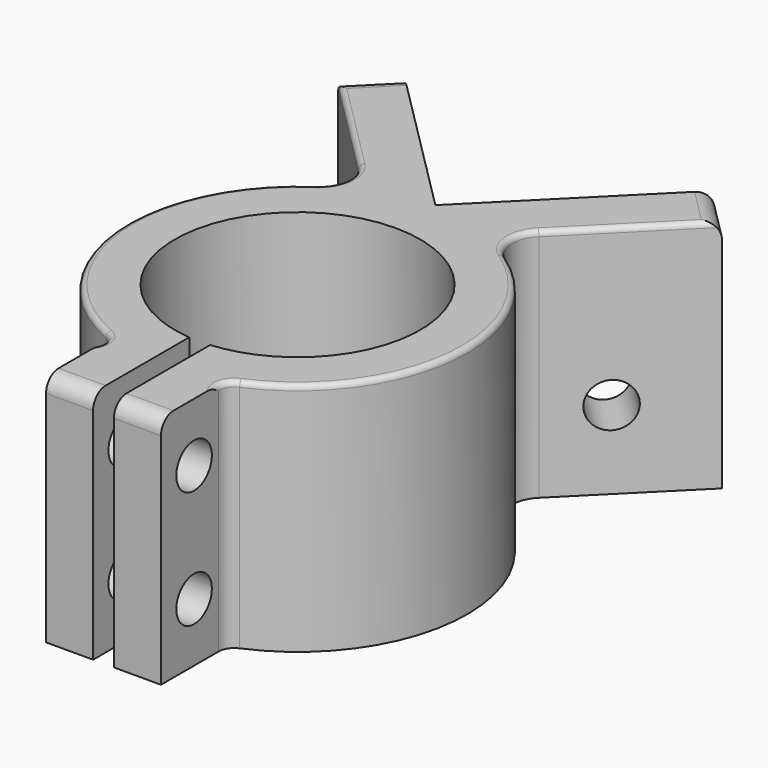
from build123d import *

# Parameters (mm, degrees)
F1_DEPTH      = 45
F2_R          = 4.25
F3_DEPTH      = 10
F4_R          = 4.25
F5_DEPTH      = 10
F6_R          = 4.25
F7_DEPTH      = 22
F9_DEPTH      = 3
F10_R         = 6
F11_T1_DEPTH  = 45
F11_T6_DEPTH  = 50.1024684741
F11_T11_DEPTH = 50.1024684741
F11_T17_DEPTH = 55.2049369483
F11_T23_DEPTH = 50.1024684741
F11_T25_DEPTH = 24
F11_T27_DEPTH = 24
F11_T29_DEPTH = 25
F11_T31_DEPTH = 25
F12_T3_ANGLE  = 122.7559288298
F12_T6_ANGLE  = 114.5305881861
F12_T9_ANGLE  = 100.9823800972
F12_T12_DEPTH = 27.0396198775
F12_T15_DEPTH = 27.0396198775
F12_T18_ANGLE = 100.9823800972
F12_T21_ANGLE = 114.5305881861
F12_T24_ANGLE = 122.7559288298


# Not quite as in the source:
# - a fillet or chamfer that OpenCascade refuses, or shapes differently, is made with other operations: its cross-section is extruded or revolved along the edge and cut away or added


with BuildPart() as f1:
    # F0 (on Top) → F1 (new body)
    with BuildSketch(Plane.XY):
        with BuildLine():
            Line((29.6984848098, 29.6984848098), (0, 0))
            Line((0, 0), (-29.6984848098, 29.6984848098))
            Line((-29.6984848098, 29.6984848098), (-36.7695526217, 22.627416998))
            Line((-36.7695526217, 22.627416998), (-11.5286496808, -2.613485943))
            ThreePointArc((-11.5286496808, -2.613485943), (-32.4987783251, -33.2817931394), (-11, -63.5818573667))
            ThreePointArc((-11, -63.5818573667), (-8.6210949019, -64.3357100238), (-6.1913611889, -64.9048122801))
            Line((-6.1913611889, -64.9048122801), (-9, -54.7082933461))
            ThreePointArc((-9, -54.7082933461), (0, -9.5), (9, -54.7082933461))
            Line((9, -54.7082933461), (6.1913611889, -64.9048122801))
            ThreePointArc((6.1913611889, -64.9048122801), (8.6210949019, -64.3357100238), (11, -63.5818573667))
            ThreePointArc((11, -63.5818573667), (32.4987783251, -33.2817931394), (11.5286496808, -2.613485943))
            Line((11.5286496808, -2.613485943), (36.7695526217, 22.627416998))
            Line((36.7695526217, 22.627416998), (29.6984848098, 29.6984848098))
        make_face()
        with BuildLine():
            ThreePointArc((-6.1913611889, -64.9048122801), (-8.6210949019, -64.3357100238), (-11, -63.5818573667))
            Line((-11, -63.5818573667), (-11, -79.4384031666))
            Line((-11, -79.4384031666), (-2, -79.4384031666))
            Line((-2, -79.4384031666), (-2, -67.4147389479))
            Line((-2, -67.4147389479), (-5.5, -67.4147389479))
            Line((-5.5, -67.4147389479), (-6.1913611889, -64.9048122801))
        make_face()
        with BuildLine():
            Line((11, -79.4384031666), (11, -63.5818573667))
            ThreePointArc((11, -63.5818573667), (8.6210949019, -64.3357100238), (6.1913611889, -64.9048122801))
            Line((6.1913611889, -64.9048122801), (5.5, -67.4147389479))
            Line((5.5, -67.4147389479), (2, -67.4147389479))
            Line((2, -67.4147389479), (2, -79.4384031666))
            Line((2, -79.4384031666), (11, -79.4384031666))
        make_face()
        with BuildLine():
            Line((-9, -54.7082933461), (-6.1913611889, -64.9048122801))
            ThreePointArc((-6.1913611889, -64.9048122801), (-4.1043610148, -65.2397925034), (-2, -65.4384031666))
            Line((-2, -65.4384031666), (-2, -56.4147389479))
            ThreePointArc((-2, -56.4147389479), (-5.565787379, -55.8313821494), (-9, -54.7082933461))
        make_face()
        with BuildLine():
            ThreePointArc((2, -65.4384031666), (4.1043610148, -65.2397925034), (6.1913611889, -64.9048122801))
            Line((6.1913611889, -64.9048122801), (9, -54.7082933461))
            ThreePointArc((9, -54.7082933461), (5.565787379, -55.8313821494), (2, -56.4147389479))
            Line((2, -56.4147389479), (2, -65.4384031666))
        make_face()
        with BuildLine():
            ThreePointArc((-2, -65.4384031666), (-4.1043610148, -65.2397925034), (-6.1913611889, -64.9048122801))
            Line((-6.1913611889, -64.9048122801), (-5.5, -67.4147389479))
            Line((-5.5, -67.4147389479), (-2, -67.4147389479))
            Line((-2, -67.4147389479), (-2, -65.4384031666))
        make_face()
        with BuildLine():
            Line((5.5, -67.4147389479), (6.1913611889, -64.9048122801))
            ThreePointArc((6.1913611889, -64.9048122801), (4.1043610148, -65.2397925034), (2, -65.4384031666))
            Line((2, -65.4384031666), (2, -67.4147389479))
            Line((2, -67.4147389479), (5.5, -67.4147389479))
        make_face()
    extrude(amount=F1_DEPTH)

    # F2 (on face) → F3 (cut, through all)
    with BuildSketch(Plane(origin=(0, 0, 0), x_dir=(-0.7071067812, -0.7071067812, 0), z_dir=(-0.7071067812, 0.7071067812, 0))):
        with Locations((-25.4, 15)):
            Circle(F2_R)
    extrude(amount=-F3_DEPTH, mode=Mode.SUBTRACT)

    # F4 (on face) → F5 (cut, through all)
    with BuildSketch(Plane(origin=(0, 0, 0), x_dir=(-0.7071067812, 0.7071067812, 0), z_dir=(0.7071067812, 0.7071067812, 0))):
        with Locations((25.4, 15)):
            Circle(F4_R)
    extrude(amount=-F5_DEPTH, mode=Mode.SUBTRACT)

    # F6 (on face) → F7 (cut, through all)
    with BuildSketch(Plane.YZ.offset(11)):
        with Locations((-71.5101302667, 33.75)):
            Circle(F6_R)
        with Locations((-71.5101302667, 11.25)):
            Circle(F6_R)
    extrude(amount=-F7_DEPTH, mode=Mode.SUBTRACT)

    # F8 (on face) → F9 (cut)
    with BuildSketch(Plane(origin=(-11, 0, 0), x_dir=(0, -1, 0), z_dir=(-1, 0, 0))):
        Polygon((78.4351302667, 37.7481506141), (71.5101302667, 41.7463012283), (64.5851302667, 37.7481506141), (64.5851302667, 29.7518493859), (71.5101302667, 25.7536987717), (78.4351302667, 29.7518493859), align=None)
        Polygon((71.5101302667, 19.2463012283), (64.5851302667, 15.2481506141), (64.5851302667, 7.2518493859), (71.5101302667, 3.2536987717), (78.4351302667, 7.2518493859), (78.4351302667, 15.2481506141), align=None)
    extrude(amount=-F9_DEPTH, mode=Mode.SUBTRACT)

    # F10
    f10_edges = [f1.edges().sort_by_distance(p)[0] for p in [
        (-11.52865, -2.613486, 22.5),
        (11.52865, -2.613486, 22.5),
    ]]
    fillet(f10_edges, radius=F10_R)

    # F11: fillet of radius 3 on 6 edges, made by hand

    # F11_s2 → F11_t1 (join)
    with BuildSketch(Plane.XY):
        with BuildLine():
            ThreePointArc((12.8169014085, -62.8659846361), (11.4950752731, -63.9719807061), (11, -65.6228447564))
            Line((11, -65.6228447564), (11, -63.5818573667))
            ThreePointArc((11, -63.5818573667), (11.9138287975, -63.2375707256), (12.8169014085, -62.8659846361))
        make_face()
    extrude(amount=F11_T1_DEPTH)


with BuildPart() as f11_tool4:
    # F11_s5 → F11_t6 (new body)
    with BuildSketch(Plane.XY):
        with BuildLine():
            ThreePointArc((-11, -65.6228447564), (-11.4950752731, -63.9719807061), (-12.8169014085, -62.8659846361))
            ThreePointArc((-12.8169014085, -62.8659846361), (-11.9138287975, -63.2375707256), (-11, -63.5818573667))
            Line((-11, -63.5818573667), (-11, -65.6228447564))
        make_face()
    extrude(amount=F11_T6_DEPTH)

    split(bisect_by=Plane(origin=(0, -19.286425463, 33.4050687982), x_dir=(1, 0, 0), z_dir=(0, 0.5, -0.8660254038)), keep=Keep.TOP)


with BuildPart() as f1_1:
    add(f1.part)

    # F11_t3: union F11_tool4
    add(f11_tool4.part)


with BuildPart() as f11_tool9:
    # F11_s10 → F11_t11 (new body)
    with BuildSketch(Plane.XY.offset(-5.1024684741)):
        with BuildLine():
            ThreePointArc((-11, -65.6228447564), (-11.4950752731, -63.9719807061), (-12.8169014085, -62.8659846361))
            ThreePointArc((-12.8169014085, -62.8659846361), (-11.9138287975, -63.2375707256), (-11, -63.5818573667))
            Line((-11, -63.5818573667), (-11, -65.6228447564))
        make_face()
    extrude(amount=F11_T11_DEPTH)

    split(bisect_by=Plane.XZ.offset(64.5851302667), keep=Keep.BOTTOM)

    split(bisect_by=Plane(origin=(0, -19.286425463, 33.4050687982), x_dir=(1, 0, 0), z_dir=(0, -0.5, 0.8660254038)), keep=Keep.TOP)


with BuildPart() as f1_2:
    add(f1_1.part)

    # F11_t8: union F11_tool9
    add(f11_tool9.part)


with BuildPart() as f11_tool15:
    # F11_s16 → F11_t17 (new body)
    with BuildSketch(Plane.XY.offset(-5.1024684741)):
        with BuildLine():
            ThreePointArc((-11, -65.6228447564), (-11.4950752731, -63.9719807061), (-12.8169014085, -62.8659846361))
            ThreePointArc((-12.8169014085, -62.8659846361), (-11.9138287975, -63.2375707256), (-11, -63.5818573667))
            Line((-11, -63.5818573667), (-11, -65.6228447564))
        make_face()
    extrude(amount=F11_T17_DEPTH)

    split(bisect_by=Plane(origin=(0, -29.0292112555, 50.2800687982), x_dir=(1, 0, 0), z_dir=(0, 0.5, -0.8660254038)), keep=Keep.TOP)

    split(bisect_by=Plane(origin=(0, -9.5436396704, -16.5300687982), x_dir=(1, 0, 0), z_dir=(0, 0.5, 0.8660254038)), keep=Keep.TOP)


with BuildPart() as f1_3:
    add(f1_2.part)

    # F11_t14: union F11_tool15
    add(f11_tool15.part)


with BuildPart() as f11_tool21:
    # F11_s22 → F11_t23 (new body)
    with BuildSketch(Plane.XY.offset(-5.1024684741)):
        with BuildLine():
            ThreePointArc((-11, -65.6228447564), (-11.4950752731, -63.9719807061), (-12.8169014085, -62.8659846361))
            ThreePointArc((-12.8169014085, -62.8659846361), (-11.9138287975, -63.2375707256), (-11, -63.5818573667))
            Line((-11, -63.5818573667), (-11, -65.6228447564))
        make_face()
    extrude(amount=F11_T23_DEPTH)

    split(bisect_by=Plane(origin=(0, 0.1991461222, 0.3449312018), x_dir=(1, 0, 0), z_dir=(0, 0.5, 0.8660254038)), keep=Keep.TOP)


with BuildPart() as f1_4:
    add(f1_3.part)

    # F11_t20: union F11_tool21
    add(f11_tool21.part)

    # F11_s26 → F11_t25 (cut)
    with BuildSketch(Plane.YZ.offset(-18.5)):
        with BuildLine():
            ThreePointArc((-76.4384031666, 45), (-78.5597235102, 44.1213203436), (-79.4384031666, 42))
            Line((-79.4384031666, 42), (-79.4384031666, 45))
            Line((-79.4384031666, 45), (-76.4384031666, 45))
        make_face()
    extrude(amount=F11_T25_DEPTH, mode=Mode.SUBTRACT)

    # F11_s28 → F11_t27 (cut)
    with BuildSketch(Plane.YZ.offset(-5.5)):
        with BuildLine():
            ThreePointArc((-76.4384031666, 45), (-78.5597235102, 44.1213203436), (-79.4384031666, 42))
            Line((-79.4384031666, 42), (-79.4384031666, 45))
            Line((-79.4384031666, 45), (-76.4384031666, 45))
        make_face()
    extrude(amount=F11_T27_DEPTH, mode=Mode.SUBTRACT)

    # F11_s30 → F11_t29 (cut)
    with BuildSketch(Plane(origin=(5.3033008589, 5.3033008589, 0), x_dir=(0, 0, 1), z_dir=(-0.7071067812, -0.7071067812, 0))):
        with BuildLine():
            ThreePointArc((45, 39), (44.1213203436, 41.1213203436), (42, 42))
            Line((42, 42), (45, 42))
            Line((45, 42), (45, 39))
        make_face()
    extrude(amount=F11_T29_DEPTH, mode=Mode.SUBTRACT)

    # F11_s32 → F11_t31 (cut)
    with BuildSketch(Plane(origin=(12.3743686708, -12.3743686708, 0), x_dir=(0, 0, 1), z_dir=(-0.7071067812, 0.7071067812, 0))):
        with BuildLine():
            ThreePointArc((45, 39), (44.1213203436, 41.1213203436), (42, 42))
            Line((42, 42), (45, 42))
            Line((45, 42), (45, 39))
        make_face()
    extrude(amount=F11_T31_DEPTH, mode=Mode.SUBTRACT)

    # F12: fillet of radius 1 on 8 edges, made by hand


with BuildPart() as f12_tool1:
    # F12_s2 → F12_t3 (revolve)
    with BuildSketch(Plane(origin=(-11.9593368598, -5.1323150169, 0), x_dir=(0, 0, 1), z_dir=(-0.9189533734, -0.3943661972, 0))):
        with BuildLine():
            ThreePointArc((44, -62.8254613228), (44.7071067812, -62.532568104), (45, -61.8254613228))
            Line((45, -61.8254613228), (45, -62.8254613228))
            Line((45, -62.8254613228), (44, -62.8254613228))
        make_face()
    revolve(axis=Axis((0, -33, 45), (0, 0, 1)), revolution_arc=F12_T3_ANGLE)


with BuildPart() as f12_tool4:
    # F12_s5 → F12_t6 (revolve)
    with BuildSketch(Plane(origin=(-11.9593368593, -5.1323150166, 0), x_dir=(0, 0, 1), z_dir=(0.9189533734, 0.3943661972, 0))):
        with BuildLine():
            ThreePointArc((44, 62.8254613229), (44.7071067812, 62.5325681041), (45, 61.8254613229))
            Line((45, 61.8254613229), (45, 62.8254613229))
            Line((45, 62.8254613229), (44, 62.8254613229))
        make_face()
    revolve(axis=Axis((14, -65.6228447564, 45), (0, 0, 1)), revolution_arc=F12_T6_ANGLE)


with BuildPart() as f12_tool7:
    # F12_s8 → F12_t9 (revolve)
    with BuildSketch(Plane(origin=(-10.2250328431, 10.2250328431, 0), x_dir=(0, 0, 1), z_dir=(-0.7071067812, 0.7071067812, 0))):
        with BuildLine():
            ThreePointArc((44, -10), (44.7071067812, -9.7071067812), (45, -9))
            Line((45, -9), (45, -10))
            Line((45, -10), (44, -10))
        make_face()
    revolve(axis=Axis((-21.5387413421, -1.0886756559, 45), (0, 0, -1)), revolution_arc=F12_T9_ANGLE)


with BuildPart() as f12_tool10:
    # F12_s11 → F12_t12 (new body)
    with BuildSketch(Plane(origin=(-29.3449314192, 29.3449314192, 0), x_dir=(0, 0, 1), z_dir=(0.7071067812, -0.7071067812, 0))):
        with BuildLine():
            ThreePointArc((44, 10), (44.7071067812, 9.7071067812), (45, 9))
            Line((45, 9), (45, 10))
            Line((45, 10), (44, 10))
        make_face()
    extrude(amount=F12_T12_DEPTH)


with BuildPart() as f12_tool13:
    # F12_s14 → F12_t15 (new body)
    with BuildSketch(Plane(origin=(10.2250328431, 10.2250328431, 0), x_dir=(0, 0, 1), z_dir=(0.7071067812, 0.7071067812, 0))):
        with BuildLine():
            ThreePointArc((44, 10), (44.7071067812, 9.7071067812), (45, 9))
            Line((45, 9), (45, 10))
            Line((45, 10), (44, 10))
        make_face()
    extrude(amount=F12_T15_DEPTH)


with BuildPart() as f12_tool16:
    # F12_s17 → F12_t18 (revolve)
    with BuildSketch(Plane(origin=(15.3023323399, -10.32840175, 0), x_dir=(0, 0, 1), z_dir=(0.8288655674, -0.5594478271, 0))):
        with BuildLine():
            ThreePointArc((44, -5.1474362764), (44.7071067812, -4.8545430576), (45, -4.1474362764))
            Line((45, -4.1474362764), (45, -5.1474362764))
            Line((45, -5.1474362764), (44, -5.1474362764))
        make_face()
    revolve(axis=Axis((21.5387413421, -1.0886756559, 45), (0, 0, -1)), revolution_arc=F12_T18_ANGLE)


with BuildPart() as f12_tool19:
    # F12_s20 → F12_t21 (revolve)
    with BuildSketch(Plane(origin=(-40.3322237445, -36.6261699102, 0), x_dir=(0, 0, 1), z_dir=(-0.74030073, -0.672275858, 0))):
        with BuildLine():
            ThreePointArc((44, -42.1687778654), (44.7071067812, -42.4616710842), (45, -43.1687778654))
            Line((45, -43.1687778654), (45, -42.1687778654))
            Line((45, -42.1687778654), (44, -42.1687778654))
        make_face()
    revolve(axis=Axis((-14, -65.6228447564, 45), (0, 0, 1)), revolution_arc=F12_T21_ANGLE)


with BuildPart() as f12_tool22:
    # F12_s23 → F12_t24 (revolve)
    with BuildSketch(Plane(origin=(-15.3023323399, -10.32840175, 0), x_dir=(0, 0, 1), z_dir=(0.8288655674, 0.5594478271, 0))):
        with BuildLine():
            ThreePointArc((44, -5.1474362764), (44.7071067812, -4.8545430576), (45, -4.1474362764))
            Line((45, -4.1474362764), (45, -5.1474362764))
            Line((45, -5.1474362764), (44, -5.1474362764))
        make_face()
    revolve(axis=Axis((0, -33, 45), (0, 0, 1)), revolution_arc=F12_T24_ANGLE)


with BuildPart() as f1_5:
    add(f1_4.part)

    # F12_t25: cut F12_tool1, F12_tool4, F12_tool7, F12_tool10, F12_tool13, F12_tool16, F12_tool19, F12_tool22
    add([f12_tool1.part, f12_tool4.part, f12_tool7.part, f12_tool10.part, f12_tool13.part, f12_tool16.part, f12_tool19.part, f12_tool22.part], mode=Mode.SUBTRACT)


solid = f1_5.part
